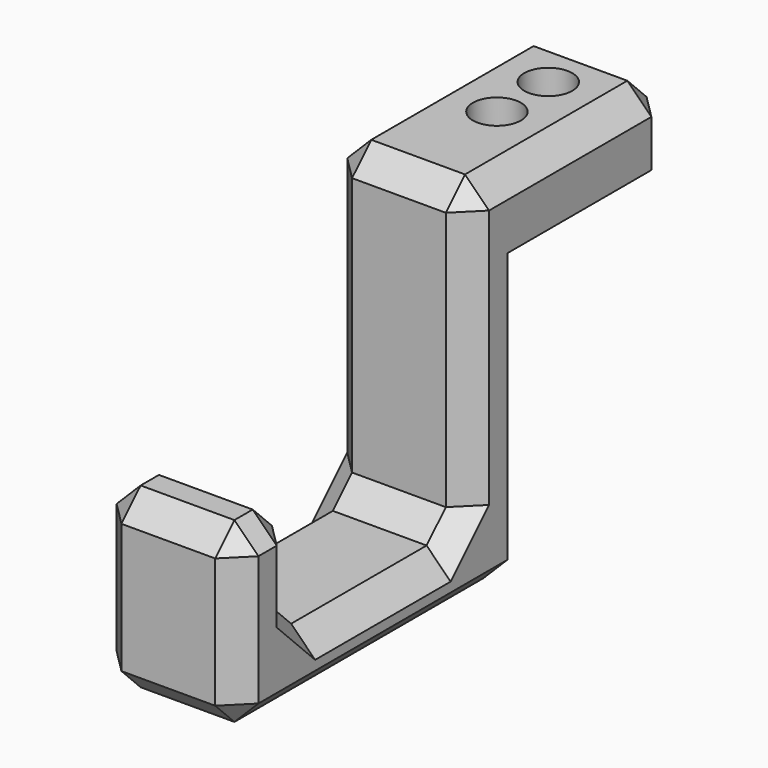
from build123d import *

# Parameters (mm, degrees)
F0_W            = 30
F0_H            = 15
F0_H_2          = 50
F0_H_3          = 25.4
F1_DEPTH        = 15
F2_DEPTH        = 38.1
F5_W            = 38.1
F5_H            = 15
F6_ANGLE        = 60
F7_DEPTH        = 61
F8_DEPTH        = 15
F9_W            = 30
F9_H            = 15
F10_DEPTH       = 25.4
F12_DEPTH       = 26.924
F14_D           = 5.08
F14_CBORE_D     = 10.16
F14_CBORE_DEPTH = 6.35
F15_D           = 5.08
F15_CBORE_D     = 10.16
F15_CBORE_DEPTH = 6.35
F17_DEPTH       = 60.96
F18_DEPTH       = 45.212
F19_SIZE        = 5.08


# Not quite as in the source:
# - a feature of the source that left no trace in its solid (it failed there, or was rolled back) is left out


with BuildPart() as f1:
    # F0 (on Front) → F1 (new body)
    with BuildSketch(Plane.XZ):
        with Locations((-21.4830274055, 50.8597951472)):
            Rectangle(F0_W, F0_H)
        with Locations((-21.4830274055, 18.3597951472)):
            Rectangle(F0_W, F0_H_2)
        with Locations((-21.4830274055, -19.3402048528)):
            Rectangle(F0_W, F0_H_3)
    extrude(amount=F1_DEPTH)

    # F0 (on Front) → F2 (join)
    with BuildSketch(Plane.XZ):
        with Locations((-21.4830274055, 50.8597951472)):
            Rectangle(F0_W, F0_H)
    extrude(amount=-F2_DEPTH)

    # F5 (on face) → F6 (revolve)
    with BuildSketch(Plane.YZ.offset(-6.4830274055)):
        with Locations((19.05, 50.8597951472)):
            Rectangle(F5_W, F5_H)
    revolve(axis=Axis((-6.4830274055, 0, 50.8597951472), (0, 0, -1)), revolution_arc=F6_ANGLE)

    # F0 (on Front) → F7 (join)
    with BuildSketch(Plane.XZ):
        with Locations((-21.4830274055, -19.3402048528)):
            Rectangle(F0_W, F0_H_3)
    extrude(amount=F7_DEPTH)

    # F8 (add): a face of the model
    f8_faces = [f1.faces().sort_by_distance(p)[0] for p in [
        (-21.4830274055, -61, -19.3402048528),
    ]]
    extrude(f8_faces, amount=F8_DEPTH)

    # F9 (on face) → F10 (join)
    with BuildSketch(Plane.XY.offset(-6.6402048528)):
        with Locations((-21.4830274055, -68.5)):
            Rectangle(F9_W, F9_H)
    extrude(amount=F10_DEPTH)

    # F11 (on face) → F12 (cut)
    with BuildSketch(Plane.XY.offset(58.3597951472)):
        with BuildLine():
            Line((-6.4830274055, 38.1), (-6.4830274055, 0))
            Line((-6.4830274055, 0), (26.5125404787, 19.05))
            ThreePointArc((26.5125404787, 19.05), (12.5669725945, 32.9955678842), (-6.4830274055, 38.1))
        make_face()
    extrude(amount=-F12_DEPTH, mode=Mode.SUBTRACT)

    # F14 (through all)
    with Locations(Plane.XY.offset(58.3597951472)):
        with Locations((-21.4830274055, 24.5092792876)):
            CounterBoreHole(F14_D / 2, F14_CBORE_D / 2, F14_CBORE_DEPTH)

    # F15 (through all)
    with Locations(Plane.XY.offset(58.3597951472)):
        with Locations((-21.4830274055, 10.9185585752)):
            CounterBoreHole(F15_D / 2, F15_CBORE_D / 2, F15_CBORE_DEPTH)

    # F16 (on face) → F17 (cut)
    with BuildSketch(Plane.YZ.offset(-6.4830274055)):
        Polygon((0, -18.8376810402), (-69.65, -18.8376810402), (-76, -18.8376810402), (-76, -32.0402048528), (0, -32.0402048528), align=None)
        Polygon((13.4356496856, -18.8376810402), (0, -18.8376810402), (0, -32.0402048528), (-76, -32.0402048528), (-76, -18.8376810402), (-82.0414423943, -18.8376810402), (-82.0414423943, -58.5641600192), (13.4356496856, -58.5641600192), align=None)
    extrude(amount=-F17_DEPTH, mode=Mode.SUBTRACT)

    # F16 (on face) → F18 (cut)
    with BuildSketch(Plane.YZ.offset(-6.4830274055)):
        Polygon((13.4356496856, -18.8376810402), (0, -18.8376810402), (0, -32.0402048528), (-76, -32.0402048528), (-76, -18.8376810402), (-82.0414423943, -18.8376810402), (-82.0414423943, -58.5641600192), (13.4356496856, -58.5641600192), align=None)
        Polygon((0, -18.8376810402), (-69.65, -18.8376810402), (-76, -18.8376810402), (-76, -32.0402048528), (0, -32.0402048528), align=None)
    extrude(amount=-F18_DEPTH, mode=Mode.SUBTRACT)

    # F19
    f19_edges = [f1.edges().sort_by_distance(p)[0] for p in [
        (-6.483027, -38, -6.640205),
        (-36.483027, -38, -6.640205),
        (-36.483027, -68.5, 18.759795),
        (-21.483027, -76, 18.759795),
        (-6.483027, -68.5, 18.759795),
        (-21.483027, -61, 18.759795),
        (-36.483027, -76, -0.038943),
        (-6.483027, -76, -0.038943),
        (-21.483027, -76, -18.837681),
        (-6.483027, -38, -18.837681),
        (-36.483027, -38, -18.837681),
        (-21.483027, 0, -18.837681),
        (-21.483027, -15, 58.359795),
        (-6.483027, -15, 25.859795),
        (-21.483027, -15, -6.640205),
        (-36.483027, -15, 25.859795),
        (-6.483027, -61, 6.059795),
        (-36.483027, -61, 6.059795),
        (-21.483027, -61, -6.640205),
        (-6.483027, 11.55, 58.359795),
        (-36.483027, 11.55, 58.359795),
        (-21.483027, 38.1, 58.359795),
        (-6.483027, 0, 12.261057),
        (-36.483027, 0, 12.261057),
        (-6.483027, 38.1, 50.859795),
        (-36.483027, 38.1, 50.859795),
    ]]
    chamfer(f19_edges, length=F19_SIZE)


solid = f1.part
